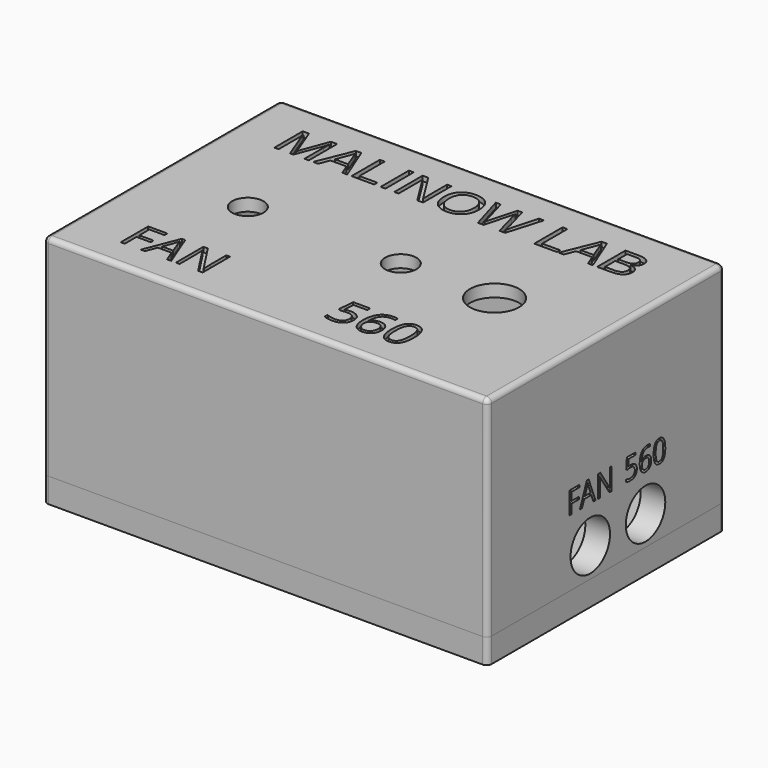
from build123d import *

# Parameters (mm, degrees)
F0_W             = 90
F0_H             = 60
F0_R             = 3.175
F0_R_2           = 5
F1_DEPTH         = 2.5
F2_W             = 90
F2_H             = 60
F2_W_2           = 80
F2_H_2           = 50
F3_DEPTH         = 40
F4_W             = 90
F4_H             = 60
F4_W_2           = 80
F4_H_2           = 50
F5_DEPTH         = 5
F7_D             = 2.4
F7_DEPTH         = 5
F7_CSINK_D       = 4
F7_CSINK_ANGLE   = 90
F7_TIP           = 0.7210327428
F7_2_D           = 2.4
F7_2_DEPTH       = 5
F7_2_CSINK_D     = 4
F7_2_CSINK_ANGLE = 90
F7_2_TIP         = 0.7210327428
F9_D             = 2.9
F9_DEPTH         = 5.2
F9_CBORE_D       = 3.7
F9_CBORE_DEPTH   = 0.2
F9_TIP           = 0.8712478976
F10_R            = 1
F10_2_R          = 1
F10_3_R          = 1
F11_R            = 5
F12_DEPTH        = 5
F13_R            = 5
F14_DEPTH        = 5
F15_TEXT_SIZE    = 10.4166666667
F16_DEPTH        = 1
F18_TEXT_SIZE    = 9.7222222222
F19_DEPTH        = 1
F20_TEXT_SIZE    = 6.25
F21_DEPTH        = 1
F22_TEXT_SIZE    = 6.25
F23_DEPTH        = 1


# Not quite as in the source:
# - a feature names something its author has since deleted; it is built from what else it names
# - Text() gives the source's letters only with a copy of the font that has no kerning and outlines rounded to 1/6400 em; it was checked with that copy


with BuildPart() as f1:
    # F0 (on Top) → F1 (new body)
    with BuildSketch(Plane.XY):
        with Locations((45, 30)):
            Rectangle(F0_W, F0_H)
        with Locations((19, 28)):
            Circle(F0_R, mode=Mode.SUBTRACT)
        with Locations((50, 28)):
            Circle(F0_R, mode=Mode.SUBTRACT)
        with Locations((69, 28)):
            Circle(F0_R_2, mode=Mode.SUBTRACT)
    extrude(amount=F1_DEPTH)

    # F10
    f10_edges = [f1.edges().sort_by_distance(p)[0] for p in [
        (45, 0, 2.5),
        (0, 30, 2.5),
        (45, 60, 2.5),
        (90, 30, 2.5),
        (0, 0, 1.25),
        (90, 0, 1.25),
        (90, 60, 1.25),
        (0, 60, 1.25),
    ]]
    fillet(f10_edges, radius=F10_R)

    # F15 (on face) → F16 (cut)
    with BuildSketch(Plane.XY.offset(2.5)):
        with Locations((8.7377929688, 46.5)):
            Text('MALINOW LAB', F15_TEXT_SIZE, font='Arimo', text_align=(TextAlign.LEFT, TextAlign.BOTTOM))
    extrude(amount=-F16_DEPTH, mode=Mode.SUBTRACT)


with BuildPart() as f3:
    # F2 (on face) → F3 (new body)
    with BuildSketch(Plane(origin=(0, 0, 0), x_dir=(1, 0, 0), z_dir=(0, 0, -1))):
        with Locations((45, -30)):
            Rectangle(F2_W, F2_H)
        with Locations((45, -30)):
            Rectangle(F2_W_2, F2_H_2, mode=Mode.SUBTRACT)
    extrude(amount=F3_DEPTH)

    # F7
    with Locations(Plane(origin=(0, 0, -45), x_dir=(1, 0, 0), z_dir=(0, 0, -1))):
        with Locations((2.5, -2.5), (2.5, -57.5), (87.5, -57.5), (87.5, -2.5)):
            CounterSinkHole(F7_D / 2, F7_CSINK_D / 2, depth=F7_DEPTH, counter_sink_angle=F7_CSINK_ANGLE)
            with Locations((0, 0, -(F7_DEPTH + F7_TIP / 2))):  # 118° drill point
                Cone(0, F7_D / 2, F7_TIP, mode=Mode.SUBTRACT)

    # F9
    with Locations(Plane(origin=(0, 0, -40), x_dir=(1, 0, 0), z_dir=(0, 0, -1))):
        with Locations((2.5, -2.5), (2.5, -57.5), (87.5, -57.5), (87.5, -2.5)):
            CounterBoreHole(F9_D / 2, F9_CBORE_D / 2, F9_CBORE_DEPTH, depth=F9_DEPTH)
            with Locations((0, 0, -(F9_DEPTH + F9_TIP / 2))):  # 118° drill point
                Cone(0, F9_D / 2, F9_TIP, mode=Mode.SUBTRACT)

    # F10#2
    f10_2_edges = [f3.edges().sort_by_distance(p)[0] for p in [
        (90, 0, -20),
        (0, 0, -20),
        (90, 60, -20),
        (0, 60, -20),
    ]]
    fillet(f10_2_edges, radius=F10_2_R)

    # F11 (on face) → F12 (cut, through all)
    with BuildSketch(Plane(origin=(0, 0, 0), x_dir=(0, -1, 0), z_dir=(-1, 0, 0))):
        with Locations((-15.5, -34)):
            Circle(F11_R)
    extrude(amount=-F12_DEPTH, mode=Mode.SUBTRACT)

    # F13 (on face) → F14 (cut, through all)
    with BuildSketch(Plane.YZ.offset(90)):
        with Locations((26, -34)):
            Circle(F13_R)
        with Locations((40, -34)):
            Circle(F13_R)
    extrude(amount=-F14_DEPTH, mode=Mode.SUBTRACT)

    # F17: union F1
    add(f1.part)

    # F18 (on face) → F19 (cut)
    with BuildSketch(Plane.XY.offset(2.5)):
        with Locations((9.9120008681, 6)):
            Text('FAN', F18_TEXT_SIZE, font='Open Sans', text_align=(TextAlign.LEFT, TextAlign.BOTTOM))
        with Locations((51.3387586806, 6)):
            Text('560', F18_TEXT_SIZE, font='Open Sans', text_align=(TextAlign.LEFT, TextAlign.BOTTOM))
    extrude(amount=-F19_DEPTH, mode=Mode.SUBTRACT)

    # F20 (on face) → F21 (cut)
    with BuildSketch(Plane.YZ.offset(90)):
        with Locations((20.1577148437, -26.5)):
            Text('FAN', F20_TEXT_SIZE, font='Open Sans', text_align=(TextAlign.LEFT, TextAlign.BOTTOM))
        with Locations((34.5927734375, -26.5)):
            Text('560', F20_TEXT_SIZE, font='Open Sans', text_align=(TextAlign.LEFT, TextAlign.BOTTOM))
    extrude(amount=-F21_DEPTH, mode=Mode.SUBTRACT)

    # F22 (on face) → F23 (cut)
    with BuildSketch(Plane(origin=(0, 0, 0), x_dir=(0, -1, 0), z_dir=(-1, 0, 0))):
        with Locations((-26.5268554687, -26.5)):
            Text('POWER', F22_TEXT_SIZE, font='Open Sans', text_align=(TextAlign.LEFT, TextAlign.BOTTOM))
    extrude(amount=-F23_DEPTH, mode=Mode.SUBTRACT)


with BuildPart() as f5:
    # F4 (on face) → F5 (new body)
    with BuildSketch(Plane(origin=(0, 0, -40), x_dir=(1, 0, 0), z_dir=(0, 0, -1))):
        with Locations((45, -30)):
            Rectangle(F4_W, F4_H)
        with Locations((45, -30)):
            Rectangle(F4_W_2, F4_H_2, mode=Mode.SUBTRACT)
        with Locations((45, -30)):
            Rectangle(F4_W_2, F4_H_2)
    extrude(amount=F5_DEPTH)

    # F7#2
    with Locations(Plane(origin=(0, 0, -45), x_dir=(1, 0, 0), z_dir=(0, 0, -1))):
        with Locations((2.5, -2.5), (2.5, -57.5), (87.5, -57.5), (87.5, -2.5)):
            CounterSinkHole(F7_2_D / 2, F7_2_CSINK_D / 2, depth=F7_2_DEPTH, counter_sink_angle=F7_2_CSINK_ANGLE)
            with Locations((0, 0, -(F7_2_DEPTH + F7_2_TIP / 2))):  # 118° drill point
                Cone(0, F7_2_D / 2, F7_2_TIP, mode=Mode.SUBTRACT)

    # F10#3
    f10_3_edges = [f5.edges().sort_by_distance(p)[0] for p in [
        (0, 60, -42.5),
        (0, 0, -42.5),
        (90, 60, -42.5),
        (90, 0, -42.5),
    ]]
    fillet(f10_3_edges, radius=F10_3_R)


solid = Compound([f3.part, f5.part])
